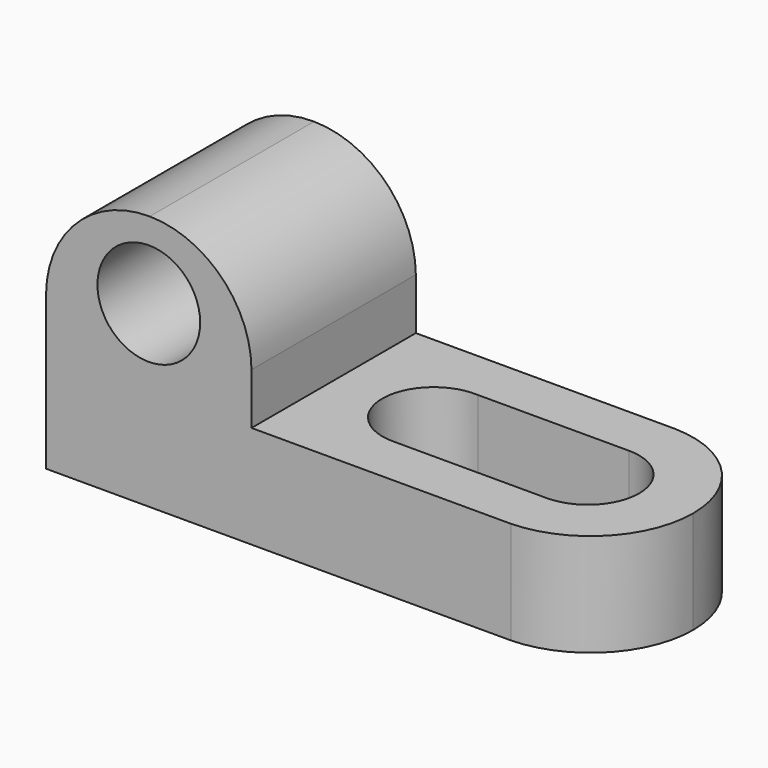
from build123d import *

# Parameters (mm, degrees)
F1_DEPTH = 25.4
F2_R     = 6.35
F3_DEPTH = 25.401
F5_DEPTH = 25.4
F7_DEPTH = 12.701
F9_DEPTH = 12.701


# Not quite as in the source:
# - ends of sketch curves that miss each other by under 0.0002 mm in the source are joined


with BuildPart() as f1:
    # F0 (on Front) → F1 (new body)
    with BuildSketch(Plane.XZ):
        Polygon((-31.4219513942, 31.5156808858), (-56.8219513942, 31.75), (-56.8219513942, 0), (13.0280486058, 0), (13.0280486058, 12.7), (-31.4219513942, 12.7), align=None)
    extrude(amount=F1_DEPTH)

    # F2 (on face) → F3 (cut, through all)
    with BuildSketch(Plane.XZ.offset(25.4)):
        with Locations((-44.1219513942, 22.1078404429)):
            Circle(F2_R)
    extrude(amount=-F3_DEPTH, mode=Mode.SUBTRACT)

    # F4 (on face) → F5 (cut)
    with BuildSketch(Plane.XZ.offset(25.4)):
        with BuildLine():
            ThreePointArc((-56.8219513942, 19.05), (-53.0189875224, 27.9952387553), (-44.0048017085, 31.6317597181))
            Line((-44.0048017085, 31.6317597181), (-56.8219513942, 31.75))
            Line((-56.8219513942, 31.75), (-56.8219513942, 19.05))
        make_face()
        with BuildLine():
            ThreePointArc((-44.0048017085, 31.6317597181), (-35.1409409401, 27.9120157755), (-31.4219513942, 19.0478384602))
            Line((-31.4219513942, 19.0478384602), (-31.4219513942, 31.5156808858))
            Line((-31.4219513942, 31.5156808858), (-44.0048017085, 31.6317597181))
        make_face()
    extrude(amount=-F5_DEPTH, mode=Mode.SUBTRACT)

    # F6 (on face) → F7 (cut, through all)
    with BuildSketch(Plane.XY.offset(12.7)):
        with BuildLine():
            ThreePointArc((-19.05, -19.05), (-14.5598719395, -17.1901280605), (-12.7, -12.7))
            ThreePointArc((-12.7, -12.7), (-14.4299815751, -8.3436334229), (-18.6773007098, -6.3609468184))
            ThreePointArc((-18.6773007098, -6.3609468184), (-25.3972627054, -12.5135699905), (-19.05, -19.05))
        make_face()
        with BuildLine():
            ThreePointArc((-18.6773007098, -6.3609468184), (-14.4299815751, -8.3436334229), (-12.7, -12.7))
            ThreePointArc((-12.7, -12.7), (-14.5598719395, -17.1901280605), (-19.05, -19.05))
            Line((-19.05, -19.05), (0, -19.05))
            ThreePointArc((0, -19.05), (4.4901280605, -17.1901280605), (6.35, -12.7))
            ThreePointArc((6.35, -12.7), (4.4901280605, -8.2098719395), (0, -6.35))
            Line((0, -6.35), (-18.6773007098, -6.3609468184))
        make_face()
    extrude(amount=-F7_DEPTH, mode=Mode.SUBTRACT)

    # F8 (on face) → F9 (cut, through all)
    with BuildSketch(Plane.XY.offset(12.7)):
        with BuildLine():
            ThreePointArc((0.6478368888, 0), (9.420896658, -3.8320853331), (13.0280486058, -12.7))
            Line((13.0280486058, -12.7), (13.0280486058, 0))
            Line((13.0280486058, 0), (0.6478368888, 0))
        make_face()
        with BuildLine():
            ThreePointArc((13.0280486058, -12.7), (9.420896658, -21.5679146669), (0.6478368888, -25.4))
            Line((0.6478368888, -25.4), (13.0280486058, -25.4))
            Line((13.0280486058, -25.4), (13.0280486058, -12.7))
        make_face()
    extrude(amount=-F9_DEPTH, mode=Mode.SUBTRACT)


solid = f1.part
